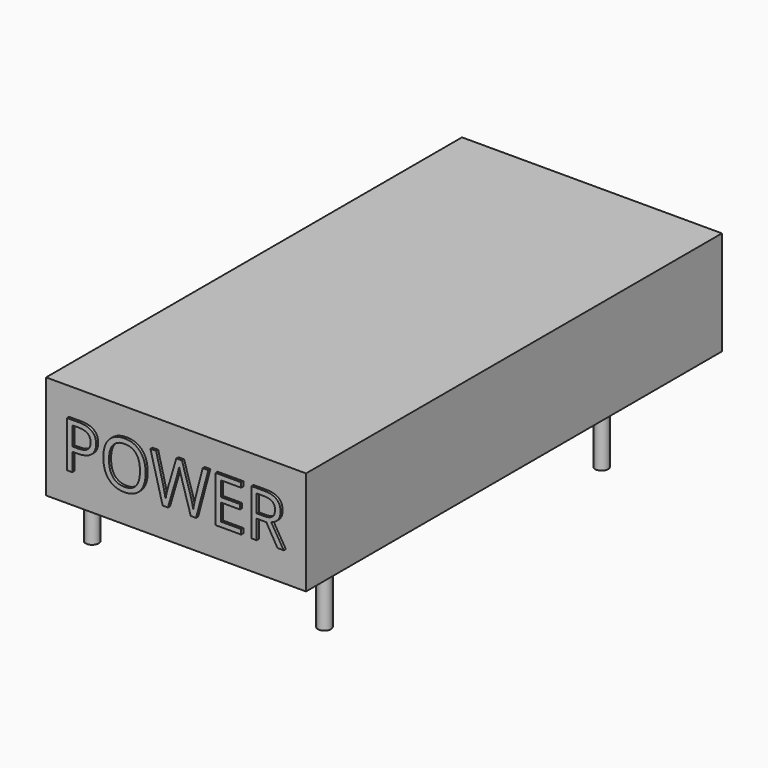
from build123d import *

# Parameters (mm, degrees)
F0_W         = 100
F0_H         = 200
F1_DEPTH     = 40
F2_TEXT_SIZE = 24.7875383745
F3_DEPTH     = 1
F4_R         = 2.5
F5_DEPTH     = 20


# Not quite as in the source:
# - Text() gives the source's letters only with a copy of the font that has no kerning and outlines rounded to 1/6400 em; it was checked with that copy


with BuildPart() as f1:
    # F0 (on Top) → F1 (new body)
    with BuildSketch(Plane.XY):
        with Locations((0, 17.8470264655)):
            Rectangle(F0_W, F0_H)
    extrude(amount=F1_DEPTH)

    # F2 (on face) → F3 (join)
    with BuildSketch(Plane.XZ.offset(82.1529735345)):
        with Locations((-43.6136640419, 11.8236504495)):
            Text('POWER', F2_TEXT_SIZE, font='Open Sans', text_align=(TextAlign.LEFT, TextAlign.BOTTOM))
    extrude(amount=F3_DEPTH)

    # F4 (on face) → F5 (join)
    with BuildSketch(Plane(origin=(0, 0, 0), x_dir=(1, 0, 0), z_dir=(0, 0, -1))):
        with Locations((-44.691182673, 66.654458642)):
            Circle(F4_R)
        with Locations((44.691182673, 66.654458642)):
            Circle(F4_R)
        with Locations((44.691182673, -66.654458642)):
            Circle(F4_R)
        with Locations((-44.691182673, -66.654458642)):
            Circle(F4_R)
    extrude(amount=F5_DEPTH)


solid = f1.part
